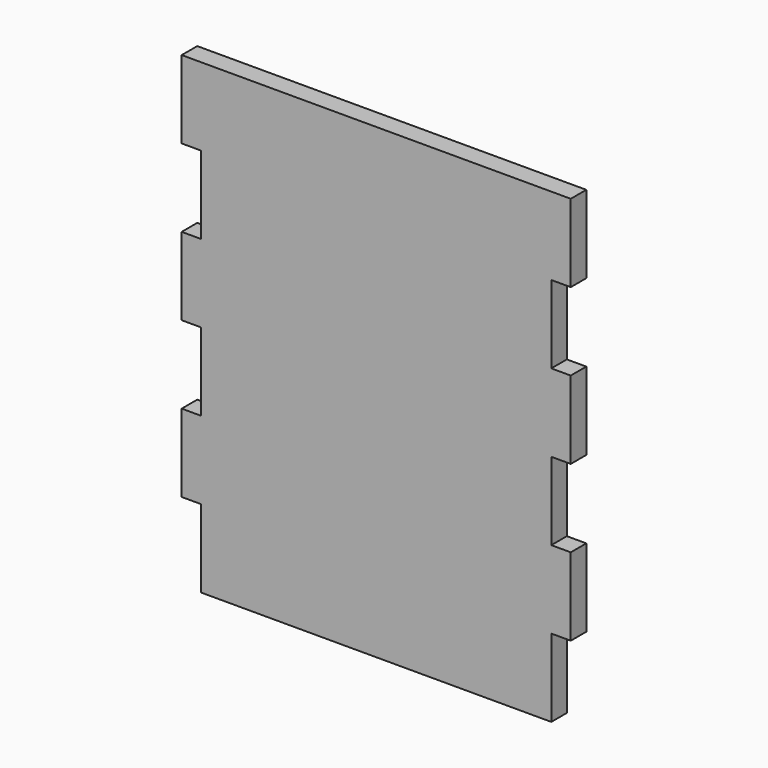
from build123d import *

# Parameters (mm, degrees)
F0_W     = 63.5
F0_H     = 76.2
F1_DEPTH = 3.175
F2_W     = 3.175
F2_H     = 12.7
F3_DEPTH = 3.176


# Not quite as in the source:
# - a pattern or mirror of a feature is missing from the dataset's text; its kind, count and spacing are read off the source's solid


with BuildPart() as f1:
    # F0 (on Front) → F1 (new body)
    with BuildSketch(Plane.XZ):
        Rectangle(F0_W, F0_H)
    extrude(amount=F1_DEPTH)

    # F2 (on Front) → F3 (cut, through all)
    with BuildSketch(Plane.XZ):
        with Locations((-30.1625, 19.05)):
            Rectangle(F2_W, F2_H)
        with Locations((-30.1625, -6.35)):
            Rectangle(F2_W, F2_H)
        with Locations((-30.1625, -31.75)):
            Rectangle(F2_W, F2_H)
    f3 = extrude(amount=F3_DEPTH, mode=Mode.SUBTRACT)

    # F3_copies: F3 across plane
    add(f3.mirror(Plane(origin=(0, 0, 0), x_dir=(0, 0, 1), z_dir=(1, 0, 0))), mode=Mode.SUBTRACT)


solid = f1.part
